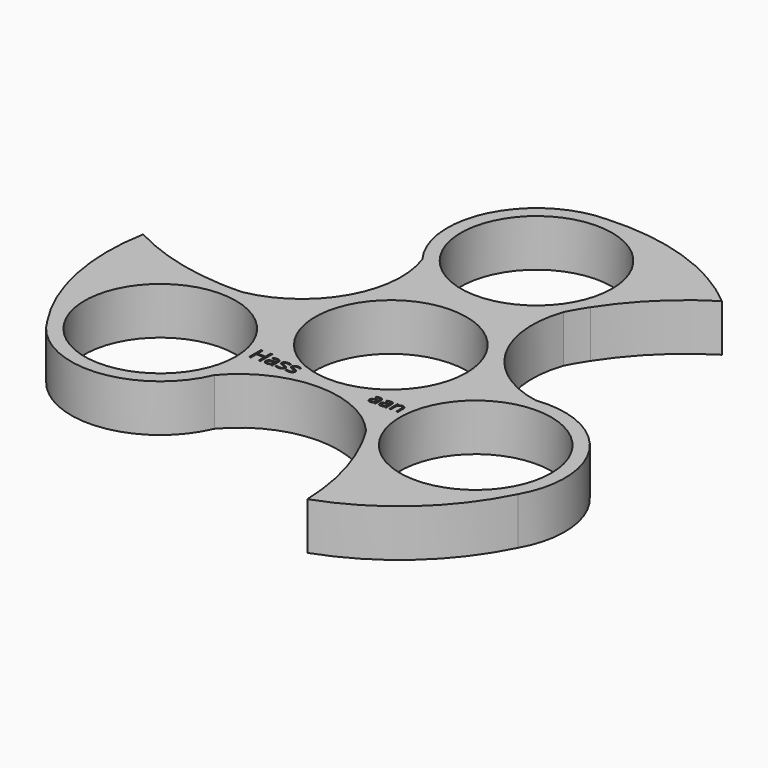
from build123d import *

# Parameters (mm, degrees)
F0_R         = 11.2
F1_DEPTH     = 7
F2_TEXT_SIZE = 3.0873436845
F3_DEPTH     = 13.4
F4_TEXT_SIZE = 2.8406800185
F5_DEPTH     = 9.9


# Not quite as in the source:
# - Text() gives the source's letters only with a copy of the font that has no kerning and outlines rounded to 1/6400 em; it was checked with that copy


with BuildPart() as f1:
    # F0 (on Top) → F1 (new body)
    with BuildSketch(Plane.XY):
        with BuildLine():
            ThreePointArc((21.7602352684, -0.3790794713), (11.6629101979, 6.6669216362), (10.4657940357, 18.9212685418))
            ThreePointArc((10.4657940357, 18.9212685418), (11.2692033032, 20.371870284), (12.1401373601, 21.7829640918))
            ThreePointArc((12.1401373601, 21.7829640918), (17.0059122311, 27.7261145683), (23.0465047061, 32.4703790247))
            ThreePointArc((23.0465047061, 32.4703790247), (12.2370493927, 38.5690257647), (-0.0710858988, 40.165152914))
            ThreePointArc((-0.0710858988, 40.165152914), (-11.8253179711, 32.8306537694), (-10.551825182, 19.0344562705))
            ThreePointArc((-10.551825182, 19.0344562705), (-11.605178601, 6.7669156953), (-21.6191962469, -0.3969907652))
            ThreePointArc((-21.6191962469, -0.3969907652), (-23.2771588402, -0.426518801), (-24.9346689532, -0.3778146866))
            ThreePointArc((-24.9346689532, -0.3778146866), (-32.5144756799, 0.8644947226), (-39.643425459, 3.7236690316))
            ThreePointArc((-39.643425459, 3.7236690316), (-39.5202808078, -8.6869172409), (-34.748499821, -20.1441386512))
            ThreePointArc((-34.748499821, -20.1441386512), (-22.5195212016, -26.6563526555), (-11.2084100865, -18.6553767991))
            ThreePointArc((-11.2084100865, -18.6553767991), (-0.0577315969, -13.4338373316), (11.1534022111, -18.5242777766))
            ThreePointArc((11.1534022111, -18.5242777766), (12.0079555369, -19.945351483), (12.7945315932, -21.4051494051))
            ThreePointArc((12.7945315932, -21.4051494051), (15.5085634488, -28.5906092908), (16.5969207529, -36.1940480563))
            ThreePointArc((16.5969207529, -36.1940480563), (27.2832314151, -29.8821085238), (34.8195857199, -20.0210142628))
            ThreePointArc((34.8195857199, -20.0210142628), (34.3448391727, -6.1743011139), (21.7602352684, -0.3790794713))
        make_face()
        with Locations((-23.352673207, -13.4826721624)):
            Circle(F0_R, mode=Mode.SUBTRACT)
        Circle(F0_R, mode=Mode.SUBTRACT)
        with Locations((23.352673207, -13.4826721624)):
            Circle(F0_R, mode=Mode.SUBTRACT)
        with Locations((0, 26.9653443247)):
            Circle(F0_R, mode=Mode.SUBTRACT)
    extrude(amount=F1_DEPTH)

    # F2 (on face) → F3 (cut)
    with BuildSketch(Plane.XY.offset(7)):
        with Locations((-11.2112455724, -12.6004500012)):
            Text('Hass', F2_TEXT_SIZE, font='Open Sans', text_align=(TextAlign.LEFT, TextAlign.BOTTOM))
    extrude(amount=-F3_DEPTH, mode=Mode.SUBTRACT)

    # F4 (on face) → F5 (cut)
    with BuildSketch(Plane.XY.offset(7)):
        with Locations((6.4620403573, -12.6233948395)):
            Text('aan', F4_TEXT_SIZE, font='Open Sans', text_align=(TextAlign.LEFT, TextAlign.BOTTOM))
    extrude(amount=-F5_DEPTH, mode=Mode.SUBTRACT)


solid = f1.part
